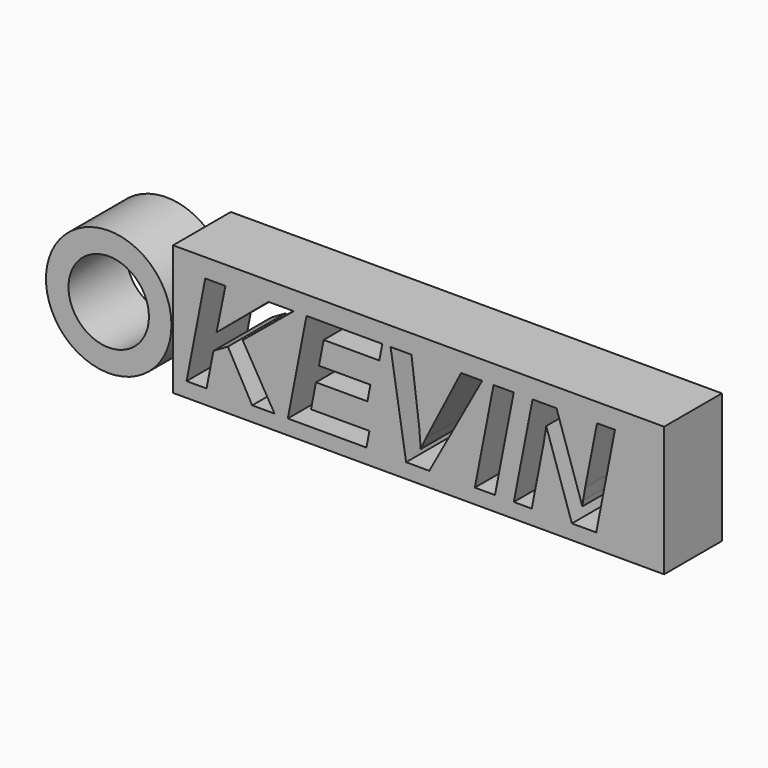
from build123d import *

# Parameters (mm, degrees)
F0_W     = 170
F0_H     = 45
F1_DEPTH = 25
F0_R     = 21.7251346757
F0_R_2   = 13.9223950692


with BuildPart() as f1:
    # F0 (on Front) → F1 (new body)
    with BuildSketch(Plane.XZ):
        with Locations((-29.2414551138, 22.5)):
            Rectangle(F0_W, F0_H)
        Polygon((-79.1214853234, 5.125280004), (-86.849139698, 5.125280004), (-95.2593150675, 20.2924132221), (-100.2568854628, 17.3803236442), (-102.6532925113, 5.125280004), (-109.5695052588, 5.125280004), (-103.1007229412, 38.5157237837), (-96.1086745277, 38.5157237837), (-99.1951861376, 23.3713412654), (-81.1842154411, 38.5157237837), (-72.4403631408, 38.5157237837), (-90.1404076064, 23.9173580612), align=None, mode=Mode.SUBTRACT)
        Polygon((-47.316006965, 5.125280004), (-74.5182603917, 5.125280004), (-68.0494780742, 38.5157237837), (-41.7951704737, 38.5157237837), (-42.8341190991, 33.116224358), (-62.1039618527, 33.116224358), (-63.7420122403, 24.7212161218), (-45.920630709, 24.7212161218), (-46.9595793344, 19.3217166961), (-64.7809608657, 19.3217166961), (-66.4872633527, 10.5323629962), (-46.2467240732, 10.5323629962), align=None, mode=Mode.SUBTRACT)
        with BuildLine():
            Line((-7.2368574362, 38.5157237837), (-25.5360036638, 5.125280004))
            Line((-25.5360036638, 5.125280004), (-33.5670007028, 5.125280004))
            Line((-33.5670007028, 5.125280004), (-38.9513329953, 38.5157237837))
            Line((-38.9513329953, 38.5157237837), (-31.7166104502, 38.5157237837))
            Line((-31.7166104502, 38.5157237837), (-29.0168607374, 17.0693974133))
            add(Edge.make_bspline(
                [(-29.0168607374, 17.0693974133), (-28.637682407, 13.5885403397), (-28.4935946414, 10.7674535611)],
                knots=[0, 0, 0, 1, 1, 1], degree=2))
            add(Edge.make_bspline(
                [(-28.4935946414, 10.7674535611), (-27.3863939165, 13.2776141087), (-26.7076647049, 14.7222835478)],
                knots=[0, 0, 0, 1, 1, 1], degree=2))
            add(Edge.make_bspline(
                [(-26.7076647049, 14.7222835478), (-26.0289354934, 16.1669529868), (-14.5398320807, 38.5157237837)],
                knots=[0, 0, 0, 1, 1, 1], degree=2))
            Line((-14.5398320807, 38.5157237837), (-7.2368574362, 38.5157237837))
        make_face(mode=Mode.SUBTRACT)
        Polygon((-2.8080545365, 5.125280004), (-9.7697686836, 5.125280004), (-3.3009863661, 38.5157237837), (3.6910620474, 38.5157237837), align=None, mode=Mode.SUBTRACT)
        with BuildLine():
            Line((32.2431903305, 5.125280004), (23.8102642613, 5.125280004))
            Line((23.8102642613, 5.125280004), (14.9450748953, 31.9256044004))
            add(Edge.make_bspline(
                [(14.9450748953, 31.9256044004), (14.3990580994, 28.0883196962), (14.0426304688, 26.26826371)],
                knots=[0, 0, 0, 1, 1, 1], degree=2))
            Line((14.0426304688, 26.26826371), (9.9171702335, 5.125280004))
            Line((9.9171702335, 5.125280004), (3.7138127473, 5.125280004))
            Line((3.7138127473, 5.125280004), (10.2053457646, 38.5157237837))
            Line((10.2053457646, 38.5157237837), (18.5017676349, 38.5157237837))
            Line((18.5017676349, 38.5157237837), (27.4352091004, 11.4803088224))
            Line((27.4352091004, 11.4803088224), (27.7158010649, 13.4217018743))
            add(Edge.make_bspline(
                [(27.7158010649, 13.4217018743), (27.9812258962, 15.385845626), (28.4059056263, 17.5471621096)],
                knots=[0, 0, 0, 1, 1, 1], degree=2))
            Line((28.4059056263, 17.5471621096), (32.5313658617, 38.5157237837))
            Line((32.5313658617, 38.5157237837), (38.7347233479, 38.5157237837))
            Line((38.7347233479, 38.5157237837), (32.2431903305, 5.125280004))
        make_face(mode=Mode.SUBTRACT)
    extrude(amount=F1_DEPTH)


with BuildPart() as f1b:
    # F0 (on Front) → F1, piece 2 (new body)
    with BuildSketch(Plane.XZ):
        with Locations((-136.5187764168, 20.501114428)):
            Circle(F0_R)
        with Locations((-136.5187764168, 20.501114428)):
            Circle(F0_R_2, mode=Mode.SUBTRACT)
    extrude(amount=F1_DEPTH)


solid = Compound([f1.part, f1b.part])
